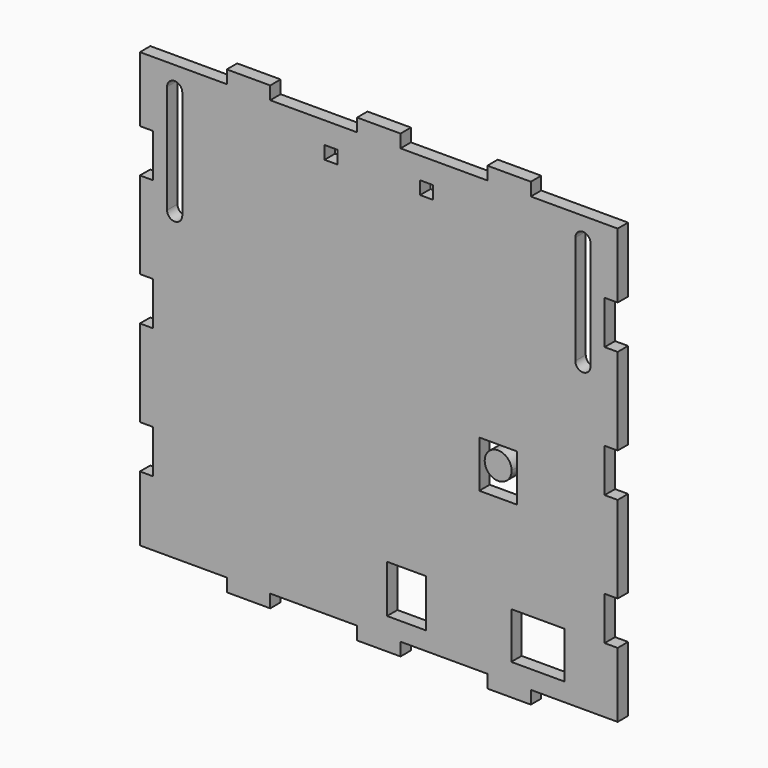
from build123d import *

# Parameters (mm, degrees)
F0_W     = 10
F0_H     = 3
F1_DEPTH = 3
F2_W     = 2.98
F2_H     = 3
F2_W_2   = 12.3
F2_H_2   = 10.7
F2_W_3   = 9
F2_H_3   = 11
F2_W_4   = 8.7
F2_H_4   = 2.2
F3_DEPTH = 25
F5_DEPTH = 25


# Not quite as in the source:
# - a feature names something its author has since deleted; it is built from what else it names


with BuildPart() as f1:
    # F0 (on Front) → F1 (new body)
    with BuildSketch(Plane.XZ):
        with Locations((30, 51.5)):
            Rectangle(F0_W, F0_H)
        with Locations((0, 51.5)):
            Rectangle(F0_W, F0_H)
        with Locations((-30, 51.5)):
            Rectangle(F0_W, F0_H)
        with Locations((30, 48.5)):
            Rectangle(F0_W, F0_H)
        with Locations((0, 48.5)):
            Rectangle(F0_W, F0_H)
        with Locations((-30, 48.5)):
            Rectangle(F0_W, F0_H)
        Polygon((55, 35), (55, 50), (35, 50), (35, 47), (25, 47), (25, 50), (5, 50), (5, 47), (-5, 47), (-5, 50), (-25, 50), (-25, 47), (-35, 47), (-35, 50), (-55, 50), (-55, 35), (-52, 35), (-52, 25), (-55, 25), (-55, 5), (-52, 5), (-52, -5), (-55, -5), (-55, -25), (-52, -25), (-52, -35), (-55, -35), (-55, -50), (-35, -50), (-35, -47), (-25, -47), (-25, -50), (-5, -50), (-5, -47), (5, -47), (5, -50), (25, -50), (25, -47), (35, -47), (35, -50), (55, -50), (55, -35), (52, -35), (52, -25), (55, -25), (55, -5), (52, -5), (52, 5), (55, 5), (55, 25), (52, 25), (52, 35), align=None)
        with Locations((30, -51.5)):
            Rectangle(F0_W, F0_H)
        with Locations((30, -48.5)):
            Rectangle(F0_W, F0_H)
        with Locations((0, -48.5)):
            Rectangle(F0_W, F0_H)
        with Locations((0, -51.5)):
            Rectangle(F0_W, F0_H)
        with Locations((-30, -48.5)):
            Rectangle(F0_W, F0_H)
        with Locations((-30, -51.5)):
            Rectangle(F0_W, F0_H)
    extrude(amount=F1_DEPTH)

    # F2 (on face) + F1_face1 (on face) → F3 (cut)
    with BuildSketch(Plane(origin=(0, 0, 0), x_dir=(-1, 0, 0), z_dir=(0, 1, 0))):
        with Locations((-11, 43.5)):
            Rectangle(F2_W, F2_H)
        with Locations((-36.65, -40.45)):
            Rectangle(F2_W_2, F2_H_2)
        with Locations((-6.4, -40.3)):
            Rectangle(F2_W_3, F2_H_3)
        with Locations((11, 43.5)):
            Rectangle(F2_W, F2_H)
        with BuildLine():
            ThreePointArc((-24.3903848411, -6.9511546684), (-24.3900962118, -6.9755765762), (-24.39, -7))
            ThreePointArc((-24.39, -7), (-27.5144234238, -10.0999037882), (-30.5896151589, -6.9511546684))
            Line((-30.5896151589, -6.9511546684), (-31.84, -6.9511546684))
            Line((-31.84, -6.9511546684), (-31.84, -11.3))
            Line((-31.84, -11.3), (-23.14, -11.3))
            Line((-23.14, -11.3), (-23.14, -6.9511546684))
            Line((-23.14, -6.9511546684), (-24.3903848411, -6.9511546684))
        make_face()
        with BuildLine():
            ThreePointArc((-30.5896151589, -6.9511546684), (-27.49, -3.9), (-24.3903848411, -6.9511546684))
            Line((-24.3903848411, -6.9511546684), (-23.14, -6.9511546684))
            Line((-23.14, -6.9511546684), (-23.14, -2.7))
            Line((-23.14, -2.7), (-31.84, -2.7))
            Line((-31.84, -2.7), (-31.84, -6.9511546684))
            Line((-31.84, -6.9511546684), (-30.5896151589, -6.9511546684))
        make_face()
        with Locations((-27.49, -12.4)):
            Rectangle(F2_W_4, F2_H_4)
    with BuildSketch(Plane.XZ.offset(3)):
        Polygon((35, 53), (25, 53), (25, 50), (5, 50), (5, 53), (-5, 53), (-5, 50), (-25, 50), (-25, 53), (-35, 53), (-35, 50), (-55, 50), (-55, 35), (-52, 35), (-52, 25), (-55, 25), (-55, 5), (-52, 5), (-52, -5), (-55, -5), (-55, -25), (-52, -25), (-52, -35), (-55, -35), (-55, -50), (-35, -50), (-35, -53), (-25, -53), (-25, -50), (-5, -50), (-5, -53), (5, -53), (5, -50), (25, -50), (25, -53), (35, -53), (35, -50), (55, -50), (55, -35), (52, -35), (52, -25), (55, -25), (55, -5), (52, -5), (52, 5), (55, 5), (55, 25), (52, 25), (52, 35), (55, 35), (55, 50), (35, 50), align=None)
    extrude(amount=-F3_DEPTH, dir=(0, 1, 0), mode=Mode.SUBTRACT)

    # F4 (on face) → F5 (cut)
    with BuildSketch(Plane.XZ.offset(3)):
        with BuildLine():
            ThreePointArc((-45.25, 45), (-47, 46.75), (-48.75, 45))
            Line((-48.75, 45), (-48.75, 20))
            ThreePointArc((-48.75, 20), (-47, 18.25), (-45.25, 20))
            Line((-45.25, 20), (-45.25, 45))
        make_face()
        with BuildLine():
            ThreePointArc((48.75, 45), (47, 46.75), (45.25, 45))
            Line((45.25, 45), (45.25, 20))
            ThreePointArc((45.25, 20), (47, 18.25), (48.75, 20))
            Line((48.75, 20), (48.75, 45))
        make_face()
    extrude(amount=-F5_DEPTH, mode=Mode.SUBTRACT)


solid = f1.part
